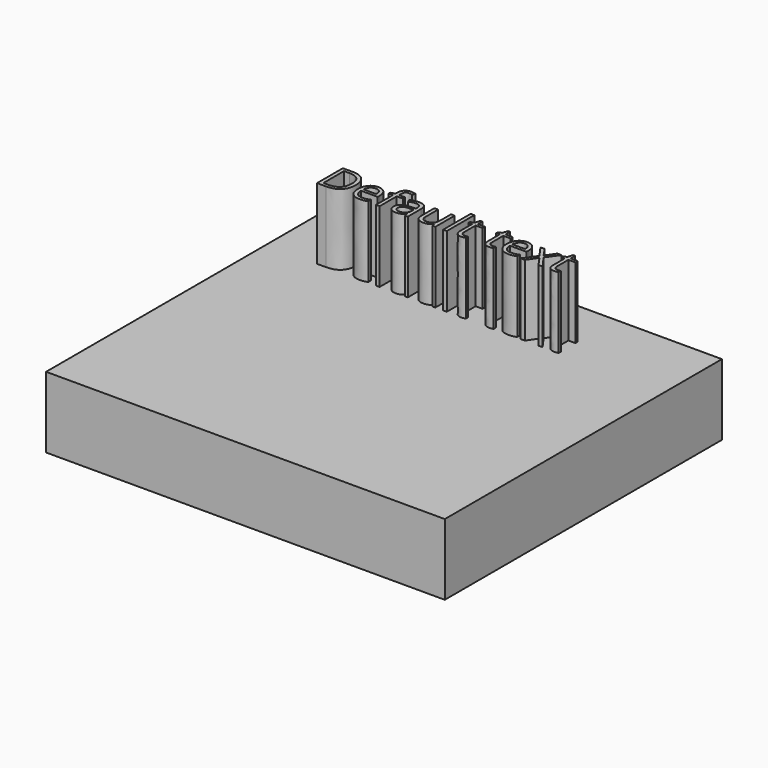
from build123d import *

# Parameters (mm, degrees)
F0_W         = 142.4828916788
F0_H         = 123.7823292613
F1_DEPTH     = 25.4
F2_TEXT_SIZE = 16.1709367401
F3_DEPTH     = 25.4


# Not quite as in the source:
# - Text() gives the source's letters only with a copy of the font that has no kerning and outlines rounded to 1/6400 em; it was checked with that copy


with BuildPart() as f1:
    # F0 (on Top) → F1 (new body)
    with BuildSketch(Plane.XY):
        with Locations((-1.7295405269, 8.8471062481)):
            Rectangle(F0_W, F0_H)
    extrude(amount=F1_DEPTH)

    # F2 (on face) → F3 (join)
    with BuildSketch(Plane.XY.offset(25.4)):
        with Locations((-56.2681593001, 45.1170951128)):
            Text('Default text', F2_TEXT_SIZE, font='Open Sans', text_align=(TextAlign.LEFT, TextAlign.BOTTOM))
    extrude(amount=F3_DEPTH)


solid = f1.part
